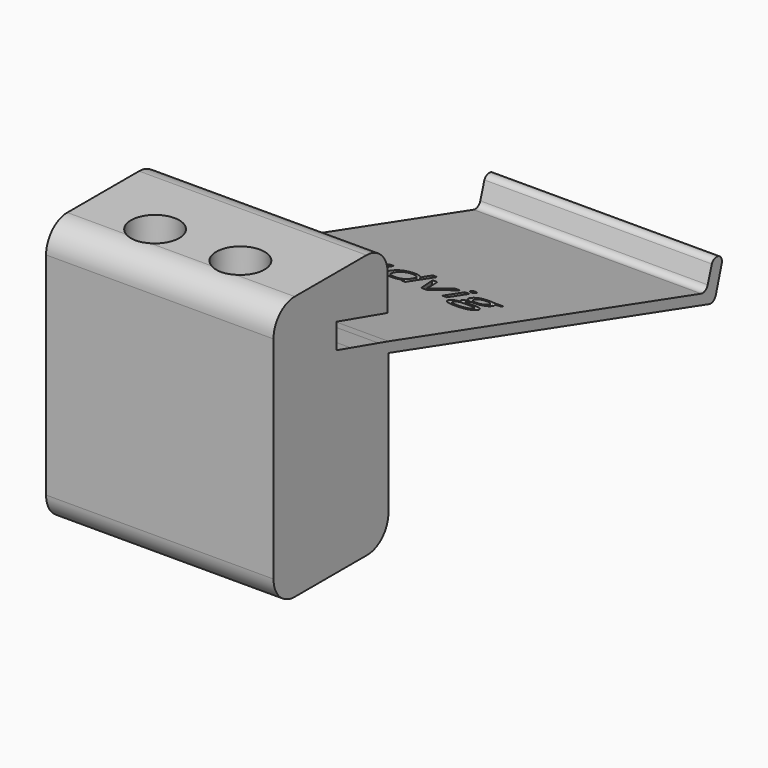
from build123d import *

# Parameters (mm, degrees)
F1_DEPTH  = 80
F4_DEPTH  = 22
F5_R      = 8.5
F6_DEPTH  = 22.5
F7_W      = 49.4286736109
F7_H      = 16.9561356306
F8_DEPTH  = 60.3
F9_W      = 1.5755122692
F9_H      = 10.3971667088
F10_DEPTH = 25


with BuildPart() as f1:
    # F0 (on Right) → F1 (new body)
    with BuildSketch(Plane.YZ):
        with BuildLine():
            ThreePointArc((-32.2318291664, 12.8581181365), (-34.9619750491, 19.4492733537), (-41.5531302664, 22.1794192365))
            Line((-41.5531302664, 22.1794192365), (-73.1118463473, 22.1794192365))
            ThreePointArc((-73.1118463473, 22.1794192365), (-79.7030015645, 19.4492733537), (-82.4331474473, 12.8581181365))
            Line((-82.4331474473, 12.8581181365), (-82.4331474473, -61.4992796635))
            ThreePointArc((-82.4331474473, -61.4992796635), (-81.2610502569, -66.0244459408), (-78.0395269394, -69.411587682))
            ThreePointArc((-78.0395269394, -69.411587682), (-76.5766946037, -70.1526882843), (-75.0066265464, -70.6259692164))
            ThreePointArc((-75.0066265464, -70.6259692164), (-74.0642204409, -70.7718002369), (-73.1118463473, -70.8205807635))
            Line((-73.1118463473, -70.8205807635), (-41.2218374732, -70.8205807635))
            ThreePointArc((-41.2218374732, -70.8205807635), (-34.6318795569, -68.0916319644), (-31.9005369883, -61.5026658346))
            Line((-31.9005369883, -61.5026658346), (-31.8690812334, -12.0527898285))
            Line((-31.8690812334, -12.0527898285), (109.1177060866, -54.2338658538))
            ThreePointArc((109.1177060866, -54.2338658538), (110.9069761748, -54.0507418606), (112.0426929702, -52.6560486304))
            Line((112.0426929702, -52.6560486304), (114.6341549506, -43.9942994883))
            ThreePointArc((114.6341549506, -43.9942994883), (114.6437769241, -42.6132673159), (113.9095705006, -41.4435308622))
            ThreePointArc((113.9095705006, -41.4435308622), (111.9034454417, -40.9732191466), (110.2978432915, -42.2646418492))
            Line((110.2978432915, -42.2646418492), (108.4831164642, -48.0129623561))
            ThreePointArc((108.4831164642, -48.0129623561), (107.3421845247, -49.382125377), (105.5685471657, -49.5568926134))
            Line((105.5685471657, -49.5568926134), (-31.8690812334, -8.4376702916))
            Line((-31.8690812334, -8.4376702916), (-36.2959507962, -7.1745254594))
            Line((-36.2959507962, -7.1745254594), (-48.491592755, -3.6946709262))
            Line((-48.491592755, -3.6946709262), (-54.7467279284, -1.9102199003))
            Line((-54.7467279284, -1.9102199003), (-54.7467279284, 6.9293941378))
            Line((-54.7467279284, 6.9293941378), (-50.4331474473, 5.6985747482))
            Line((-50.4331474473, 5.6985747482), (-46.4961274784, 4.5752015931))
            Line((-46.4961274784, 4.5752015931), (-32.2318291664, 0.5050851276))
            Line((-32.2318291664, 0.5050851276), (-32.2318291664, 12.8581181365))
        make_face()
    extrude(amount=F1_DEPTH)

    # F3 (on face) → F4 (cut)
    with BuildSketch(Plane(origin=(0, -54.7467279284, 0), x_dir=(-1, 0, 0), z_dir=(0, 1, 0))):
        Polygon((-71, 5.1884208806), (-71, 2.5095871187), (-71, 0), (-9, 0), (-9, 5.1884208806), (-69.0773031712, 5.1884208806), align=None)
    extrude(amount=-F4_DEPTH, mode=Mode.SUBTRACT)

    # F5 (on face) → F6 (cut)
    with BuildSketch(Plane(origin=(0, 0, 5.1884208806), x_dir=(1, 0, 0), z_dir=(0, 0, -1))):
        with Locations((55, 65.7467279284)):
            Circle(F5_R)
        with Locations((25, 65.7467279284)):
            Circle(F5_R)
    extrude(amount=-F6_DEPTH, mode=Mode.SUBTRACT)

    # F7 (on face) → F8 (cut)
    with BuildSketch(Plane.XY):
        with Locations((38.2213593278, -65.6192749739)):
            Rectangle(F7_W, F7_H)
    extrude(amount=-F8_DEPTH, mode=Mode.SUBTRACT)

    # F9 (on face) → F10 (cut)
    with BuildSketch(Plane(origin=(0, -4.9353020431, -16.4958423322), x_dir=(1, 0, 0), z_dir=(0, 0.286631123, 0.9580410217))):
        with BuildLine():
            Line((68.1775680531, 38.9351487613), (68.1775680531, 39.9308482301))
            Line((68.1775680531, 39.9308482301), (64.5833358245, 39.9308482301))
            add(Edge.make_bspline(
                [(63.1110363051, 40.1220953841), (63.9276312963, 40.1220953841), (64.5833358245, 39.9308482301)],
                knots=[0, 0, 0, 1, 1, 1], degree=2))
            add(Edge.make_bspline(
                [(60.2104544685, 39.1962163049), (61.2349927939, 40.1220953841), (63.1110363051, 40.1220953841)],
                knots=[0, 0, 0, 1, 1, 1], degree=2))
            add(Edge.make_bspline(
                [(59.1859161432, 36.5642911848), (59.1859161432, 38.2703372258), (60.2104544685, 39.1962163049)],
                knots=[0, 0, 0, 1, 1, 1], degree=2))
            add(Edge.make_bspline(
                [(59.6928728849, 34.741371883), (59.1859161432, 35.5382350249), (59.1859161432, 36.5642911848)],
                knots=[0, 0, 0, 1, 1, 1], degree=2))
            add(Edge.make_bspline(
                [(61.0073176104, 33.6136208078), (60.1998296266, 33.9445087411), (59.6928728849, 34.741371883)],
                knots=[0, 0, 0, 1, 1, 1], degree=2))
            add(Edge.make_bspline(
                [(60.048046171, 32.7879188094), (60.3516130822, 33.2159481542), (61.0073176104, 33.6136208078)],
                knots=[0, 0, 0, 1, 1, 1], degree=2))
            add(Edge.make_bspline(
                [(59.7444792598, 31.7922193406), (59.7444792598, 32.3598894646), (60.048046171, 32.7879188094)],
                knots=[0, 0, 0, 1, 1, 1], degree=2))
            add(Edge.make_bspline(
                [(60.0146538108, 30.908839629), (59.7444792598, 31.288298268), (59.7444792598, 31.7922193406)],
                knots=[0, 0, 0, 1, 1, 1], degree=2))
            add(Edge.make_bspline(
                [(60.6825010155, 30.3502765124), (60.2848283618, 30.52938099), (60.0146538108, 30.908839629)],
                knots=[0, 0, 0, 1, 1, 1], degree=2))
            add(Edge.make_bspline(
                [(58.9764549745, 29.4107369222), (59.5835887969, 30.1043873143), (60.6825010155, 30.3502765124)],
                knots=[0, 0, 0, 1, 1, 1], degree=2))
            add(Edge.make_bspline(
                [(58.3693211521, 27.7699577671), (58.3693211521, 28.7170865301), (58.9764549745, 29.4107369222)],
                knots=[0, 0, 0, 1, 1, 1], degree=2))
            add(Edge.make_bspline(
                [(59.4743047089, 25.6237397049), (58.3693211521, 26.3826569829), (58.3693211521, 27.7699577671)],
                knots=[0, 0, 0, 1, 1, 1], degree=2))
            add(Edge.make_bspline(
                [(62.619257909, 24.8648224269), (60.5792882656, 24.8648224269), (59.4743047089, 25.6237397049)],
                knots=[0, 0, 0, 1, 1, 1], degree=2))
            add(Edge.make_bspline(
                [(66.6597334971, 25.7709696568), (65.275468382, 24.8648224269), (62.619257909, 24.8648224269)],
                knots=[0, 0, 0, 1, 1, 1], degree=2))
            add(Edge.make_bspline(
                [(68.0439986122, 28.4044126115), (68.0439986122, 26.6771168868), (66.6597334971, 25.7709696568)],
                knots=[0, 0, 0, 1, 1, 1], degree=2))
            add(Edge.make_bspline(
                [(67.1393692168, 30.4732211114), (68.0439986122, 29.7613567046), (68.0439986122, 28.4044126115)],
                knots=[0, 0, 0, 1, 1, 1], degree=2))
            add(Edge.make_bspline(
                [(64.543872126, 31.1850855182), (66.2347398214, 31.1850855182), (67.1393692168, 30.4732211114)],
                knots=[0, 0, 0, 1, 1, 1], degree=2))
            Line((64.543872126, 31.1850855182), (62.7042566441, 31.1850855182))
            add(Edge.make_bspline(
                [(61.5006138412, 31.3884753487), (61.8512336236, 31.1850855182), (62.7042566441, 31.1850855182)],
                knots=[0, 0, 0, 1, 1, 1], degree=2))
            add(Edge.make_bspline(
                [(61.1499940587, 32.019894524), (61.1499940587, 31.5918651792), (61.5006138412, 31.3884753487)],
                knots=[0, 0, 0, 1, 1, 1], degree=2))
            add(Edge.make_bspline(
                [(62.1548005348, 33.3555889333), (61.1499940587, 32.8243468387), (61.1499940587, 32.019894524)],
                knots=[0, 0, 0, 1, 1, 1], degree=2))
            add(Edge.make_bspline(
                [(63.02603757, 33.2796972055), (62.5615801958, 33.2796972055), (62.1548005348, 33.3555889333)],
                knots=[0, 0, 0, 1, 1, 1], degree=2))
            add(Edge.make_bspline(
                [(65.8917092118, 34.1903979391), (64.8474390372, 33.2796972055), (63.02603757, 33.2796972055)],
                knots=[0, 0, 0, 1, 1, 1], degree=2))
            add(Edge.make_bspline(
                [(66.9359793863, 36.6310759052), (66.9359793863, 35.1010986728), (65.8917092118, 34.1903979391)],
                knots=[0, 0, 0, 1, 1, 1], degree=2))
            add(Edge.make_bspline(
                [(66.7265182176, 37.8392722118), (66.9359793863, 37.301958779), (66.9359793863, 36.6310759052)],
                knots=[0, 0, 0, 1, 1, 1], degree=2))
            add(Edge.make_bspline(
                [(66.2529538361, 38.7074735779), (66.5170570488, 38.3765856447), (66.7265182176, 37.8392722118)],
                knots=[0, 0, 0, 1, 1, 1], degree=2))
            Line((66.2529538361, 38.7074735779), (68.1775680531, 38.9351487613))
        make_face()
        with BuildLine():
            Line((58.4288015962, 28.3339321613), (58.4874711931, 28.3339321613))
            Line((58.4874711931, 28.3339321613), (59.9432890305, 28.3339321613))
            add(Edge.make_bspline(
                [(60.4851825232, 29.2589534666), (60.0703747901, 28.9041559893), (59.9432890305, 28.3339321613)],
                knots=[0, 0, 0, 0.6936273134, 0.6936273134, 0.6936273134], degree=2))
            add(Edge.make_bspline(
                [(62.1548005348, 29.770463712), (61.0832093382, 29.770463712), (60.4851825232, 29.2589534666)],
                knots=[0, 0, 0, 1, 1, 1], degree=2))
            Line((62.1548005348, 29.770463712), (64.0429867225, 29.770463712))
            add(Edge.make_bspline(
                [(66.0055468035, 29.4426114479), (65.4849295507, 29.770463712), (64.0429867225, 29.770463712)],
                knots=[0, 0, 0, 1, 1, 1], degree=2))
            add(Edge.make_bspline(
                [(66.5254195492, 28.3339321613), (66.5064764157, 29.1271572314), (66.0055468035, 29.4426114479)],
                knots=[0.0378159586, 0.0378159586, 0.0378159586, 1, 1, 1], degree=2))
            Line((66.5254195492, 28.3339321613), (67.9926872253, 28.3339321613))
            Line((67.9926872253, 28.3339321613), (68.0369660258, 28.3339321613))
            Line((68.0369660258, 28.3339321613), (68.0369660258, 28.2860677689))
            Line((68.0369660258, 28.2860677689), (68.0369660258, 28.1646177173))
            Line((68.0369660258, 28.1646177173), (68.034209311, 28.1332600862))
            Line((68.034209311, 28.1332600862), (66.5219728583, 28.1382272438))
            add(Edge.make_bspline(
                [(65.572963955, 26.6634563758), (66.4629576461, 27.2175766516), (66.5219728583, 28.1382272438)],
                knots=[0, 0, 0, 0.9336903028, 0.9336903028, 0.9336903028], degree=2))
            add(Edge.make_bspline(
                [(62.6374719236, 26.0699830644), (64.6197638538, 26.0699830644), (65.572963955, 26.6634563758)],
                knots=[0, 0, 0, 1, 1, 1], degree=2))
            add(Edge.make_bspline(
                [(60.5990201149, 26.5071194165), (61.3108845217, 26.0699830644), (62.6374719236, 26.0699830644)],
                knots=[0, 0, 0, 1, 1, 1], degree=2))
            add(Edge.make_bspline(
                [(59.8871557081, 27.7881717818), (59.8871557081, 26.9442557686), (60.5990201149, 26.5071194165)],
                knots=[0, 0, 0, 1, 1, 1], degree=2))
            add(Edge.make_bspline(
                [(59.9119054363, 28.1599389586), (59.8871557081, 27.9833208141), (59.8871557081, 27.7881717818)],
                knots=[0.7965653679, 0.7965653679, 0.7965653679, 1, 1, 1], degree=2))
            Line((59.9119054363, 28.1599389586), (58.4874711931, 28.1646177173))
            Line((58.4874711931, 28.1646177173), (58.3997890353, 28.1646177173))
            Line((58.3997890353, 28.1646177173), (58.3997890353, 28.180770576))
            Line((58.3997890353, 28.180770576), (58.417674154, 28.2701700926))
            Line((58.417674154, 28.2701700926), (58.4288015962, 28.3339321613))
        make_face(mode=Mode.SUBTRACT)
        with BuildLine():
            add(Edge.make_bspline(
                [(60.7401787286, 36.6007192141), (60.7401787286, 35.5109140029), (61.3564195583, 34.9508330517)],
                knots=[0, 0, 0, 1, 1, 1], degree=2))
            add(Edge.make_bspline(
                [(61.3382055437, 38.3750678101), (60.7401787286, 37.7785588296), (60.7401787286, 36.6007192141)],
                knots=[0, 0, 0, 1, 1, 1], degree=2))
            add(Edge.make_bspline(
                [(63.0472872538, 38.9715767906), (61.9362323587, 38.9715767906), (61.3382055437, 38.3750678101)],
                knots=[0, 0, 0, 1, 1, 1], degree=2))
            add(Edge.make_bspline(
                [(65.3786811318, 36.6310759052), (65.3786811318, 38.9715767906), (63.0472872538, 38.9715767906)],
                knots=[0, 0, 0, 1, 1, 1], degree=2))
            add(Edge.make_bspline(
                [(63.0746082758, 34.3907521005), (65.3786811318, 34.3907521005), (65.3786811318, 36.6310759052)],
                knots=[0, 0, 0, 1, 1, 1], degree=2))
            add(Edge.make_bspline(
                [(61.3564195583, 34.9508330517), (61.9726603881, 34.3907521005), (63.0746082758, 34.3907521005)],
                knots=[0, 0, 0, 1, 1, 1], degree=2))
        make_face(mode=Mode.SUBTRACT)
        with BuildLine():
            Line((40.1067357739, 30.9270536437), (40.191734509, 30.9270536437))
            Line((40.191734509, 30.9270536437), (40.4011956777, 29.5336815212))
            Line((40.4011956777, 29.5336815212), (41.682248043, 29.5336815212))
            Line((41.682248043, 29.5336815212), (41.682248043, 44.2961404132))
            Line((41.682248043, 44.2961404132), (40.1067357739, 44.2961404132))
            Line((40.1067357739, 44.2961404132), (40.1067357739, 40.064417671))
            Line((40.1067357739, 40.064417671), (40.1461994723, 39.332821415))
            Line((40.1461994723, 39.332821415), (40.2129841928, 38.5830111443))
            Line((40.2129841928, 38.5830111443), (40.0885217592, 38.5830111443))
            add(Edge.make_bspline(
                [(36.8433914784, 40.1220953841), (38.9592528495, 40.1220953841), (40.0885217592, 38.5830111443)],
                knots=[0, 0, 0, 1, 1, 1], degree=2))
            add(Edge.make_bspline(
                [(33.6741529254, 38.6983665706), (34.8125288424, 40.1220953841), (36.8433914784, 40.1220953841)],
                knots=[0, 0, 0, 1, 1, 1], degree=2))
            add(Edge.make_bspline(
                [(32.5357770084, 34.7034260191), (32.5357770084, 37.274637757), (33.6741529254, 38.6983665706)],
                knots=[0, 0, 0, 1, 1, 1], degree=2))
            add(Edge.make_bspline(
                [(33.6695994217, 30.7373243242), (32.5357770084, 32.1322142812), (32.5357770084, 34.7034260191)],
                knots=[0, 0, 0, 1, 1, 1], degree=2))
            add(Edge.make_bspline(
                [(36.8433914784, 29.3424343672), (34.8034218351, 29.3424343672), (33.6695994217, 30.7373243242)],
                knots=[0, 0, 0, 1, 1, 1], degree=2))
            add(Edge.make_bspline(
                [(40.1067357739, 30.9270536437), (39.0169305626, 29.3424343672), (36.8433914784, 29.3424343672)],
                knots=[0, 0, 0, 1, 1, 1], degree=2))
        make_face()
        with BuildLine():
            add(Edge.make_bspline(
                [(37.0437456398, 30.6629504309), (38.6556859383, 30.6629504309), (39.3812108561, 31.5402588043)],
                knots=[0, 0, 0, 1, 1, 1], degree=2))
            add(Edge.make_bspline(
                [(34.8990454121, 31.6783817489), (35.6291238336, 30.6629504309), (37.0437456398, 30.6629504309)],
                knots=[0, 0, 0, 1, 1, 1], degree=2))
            add(Edge.make_bspline(
                [(34.1689669907, 34.6852120044), (34.1689669907, 32.6938130669), (34.8990454121, 31.6783817489)],
                knots=[0, 0, 0, 1, 1, 1], degree=2))
            add(Edge.make_bspline(
                [(34.9035989158, 37.7254346201), (34.1689669907, 36.6492899199), (34.1689669907, 34.6852120044)],
                knots=[0, 0, 0, 1, 1, 1], degree=2))
            add(Edge.make_bspline(
                [(37.0255316251, 38.8015793204), (35.6382308409, 38.8015793204), (34.9035989158, 37.7254346201)],
                knots=[0, 0, 0, 1, 1, 1], degree=2))
            add(Edge.make_bspline(
                [(39.3721038487, 37.8574862265), (38.6374719236, 38.8015793204), (37.0255316251, 38.8015793204)],
                knots=[0, 0, 0, 1, 1, 1], degree=2))
            add(Edge.make_bspline(
                [(40.1067357739, 34.7034260191), (40.1067357739, 36.9133931327), (39.3721038487, 37.8574862265)],
                knots=[0, 0, 0, 1, 1, 1], degree=2))
            Line((40.1067357739, 34.7034260191), (40.1067357739, 34.3725380859))
            add(Edge.make_bspline(
                [(39.3812108561, 31.5402588043), (40.1067357739, 32.4175671777), (40.1067357739, 34.3725380859)],
                knots=[0, 0, 0, 1, 1, 1], degree=2))
        make_face(mode=Mode.SUBTRACT)
        with BuildLine():
            Line((22.6728880633, 33.185591463), (22.6728880633, 39.9308482301))
            Line((22.6728880633, 39.9308482301), (21.0791617794, 39.9308482301))
            Line((21.0791617794, 39.9308482301), (21.0791617794, 33.1279137499))
            add(Edge.make_bspline(
                [(22.0217370387, 30.2440280935), (21.0791617794, 31.1456218197), (21.0791617794, 33.1279137499)],
                knots=[0, 0, 0, 1, 1, 1], degree=2))
            add(Edge.make_bspline(
                [(24.8616054931, 29.3424343672), (22.964312298, 29.3424343672), (22.0217370387, 30.2440280935)],
                knots=[0, 0, 0, 1, 1, 1], degree=2))
            add(Edge.make_bspline(
                [(26.8226477395, 29.7507318627), (25.9635533807, 29.3424343672), (24.8616054931, 29.3424343672)],
                knots=[0, 0, 0, 1, 1, 1], degree=2))
            add(Edge.make_bspline(
                [(28.164413487, 30.9270536437), (27.6817420982, 30.1590293583), (26.8226477395, 29.7507318627)],
                knots=[0, 0, 0, 1, 1, 1], degree=2))
            Line((28.164413487, 30.9270536437), (28.2494122221, 30.9270536437))
            Line((28.2494122221, 30.9270536437), (28.4770874055, 29.5336815212))
            Line((28.4770874055, 29.5336815212), (29.7763537855, 29.5336815212))
            Line((29.7763537855, 29.5336815212), (29.7763537855, 39.9308482301))
            Line((29.7763537855, 39.9308482301), (28.2008415163, 39.9308482301))
            Line((28.2008415163, 39.9308482301), (28.2008415163, 34.4666438283))
            add(Edge.make_bspline(
                [(27.4479955765, 31.5539193153), (28.2008415163, 32.4448881997), (28.2008415163, 34.4666438283)],
                knots=[0, 0, 0, 1, 1, 1], degree=2))
            add(Edge.make_bspline(
                [(25.0619596545, 30.6629504309), (26.6951496368, 30.6629504309), (27.4479955765, 31.5539193153)],
                knots=[0, 0, 0, 1, 1, 1], degree=2))
            add(Edge.make_bspline(
                [(23.2511830291, 31.288298268), (23.829477995, 30.6629504309), (25.0619596545, 30.6629504309)],
                knots=[0, 0, 0, 1, 1, 1], degree=2))
            add(Edge.make_bspline(
                [(22.6728880633, 33.185591463), (22.6728880633, 31.9136461051), (23.2511830291, 31.288298268)],
                knots=[0, 0, 0, 1, 1, 1], degree=2))
        make_face()
        with BuildLine():
            Line((43.3518660547, 39.9308482301), (47.2982359004, 29.5336815212))
            Line((47.2982359004, 29.5336815212), (49.1378513823, 29.5336815212))
            Line((49.1378513823, 29.5336815212), (53.084221228, 39.9308482301))
            Line((53.084221228, 39.9308482301), (51.3963892016, 39.9308482301))
            add(Edge.make_bspline(
                [(48.9071405297, 33.0383615111), (49.4626679773, 34.6184272839), (51.3963892016, 39.9308482301)],
                knots=[0, 0, 0, 1, 1, 1], degree=2))
            add(Edge.make_bspline(
                [(48.2484003324, 30.9574103348), (48.3516130822, 31.4582957383), (48.9071405297, 33.0383615111)],
                knots=[0, 0, 0, 1, 1, 1], degree=2))
            Line((48.2484003324, 30.9574103348), (48.1725086046, 30.9574103348))
            add(Edge.make_bspline(
                [(47.2800218857, 33.7654042635), (48.0389391637, 31.6009721865), (48.1725086046, 30.9574103348)],
                knots=[0, 0, 0, 1, 1, 1], degree=2))
            Line((47.2800218857, 33.7654042635), (45.039698081, 39.9308482301))
            Line((45.039698081, 39.9308482301), (43.3518660547, 39.9308482301))
        make_face()
        Polygon((11.343770937, 43.4036536943), (11.343770937, 29.5336815212), (19.0756201655, 29.5336815212), (19.0756201655, 30.9938383641), (12.9557112355, 30.9938383641), (12.9557112355, 43.4036536943), align=None)
        with Locations((55.5415953742, 34.7322648756)):
            Rectangle(F9_W, F9_H)
        with BuildLine():
            add(Edge.make_bspline(
                [(54.6202697987, 42.7479491661), (54.6202697987, 43.288298268), (54.885890846, 43.5402588043)],
                knots=[0, 0, 0, 1, 1, 1], degree=2))
            add(Edge.make_bspline(
                [(54.885890846, 41.9556395278), (54.6202697987, 42.2167070714), (54.6202697987, 42.7479491661)],
                knots=[0, 0, 0, 1, 1, 1], degree=2))
            add(Edge.make_bspline(
                [(55.5522202161, 41.6945719842), (55.1515118933, 41.6945719842), (54.885890846, 41.9556395278)],
                knots=[0, 0, 0, 1, 1, 1], degree=2))
            add(Edge.make_bspline(
                [(56.2064069097, 41.9556395278), (55.9316788551, 41.6945719842), (55.5522202161, 41.6945719842)],
                knots=[0, 0, 0, 1, 1, 1], degree=2))
            add(Edge.make_bspline(
                [(56.4811349644, 42.7479491661), (56.4811349644, 42.2167070714), (56.2064069097, 41.9556395278)],
                knots=[0, 0, 0, 1, 1, 1], degree=2))
            add(Edge.make_bspline(
                [(56.2064069097, 43.5357053006), (56.4811349644, 43.2791912607), (56.4811349644, 42.7479491661)],
                knots=[0, 0, 0, 1, 1, 1], degree=2))
            add(Edge.make_bspline(
                [(55.5522202161, 43.7922193406), (55.9316788551, 43.7922193406), (56.2064069097, 43.5357053006)],
                knots=[0, 0, 0, 1, 1, 1], degree=2))
            add(Edge.make_bspline(
                [(54.885890846, 43.5402588043), (55.1515118933, 43.7922193406), (55.5522202161, 43.7922193406)],
                knots=[0, 0, 0, 1, 1, 1], degree=2))
        make_face()
        with BuildLine():
            Line((67.9926872253, 28.3339321613), (66.5254195492, 28.3339321613))
            add(Edge.make_bspline(
                [(66.5261640562, 28.2708431706), (66.5261640562, 28.3027566636), (66.5254195492, 28.3339321613)],
                knots=[0, 0, 0, 0.0378159586, 0.0378159586, 0.0378159586], degree=2))
            add(Edge.make_bspline(
                [(66.5219728583, 28.1382272438), (66.5261640562, 28.2036108745), (66.5261640562, 28.2708431706)],
                knots=[0.9336903028, 0.9336903028, 0.9336903028, 1, 1, 1], degree=2))
            Line((66.5219728583, 28.1382272438), (68.034209311, 28.1332600862))
            Line((68.034209311, 28.1332600862), (68.0369660258, 28.1646177173))
            Line((68.0369660258, 28.1646177173), (68.0369660258, 28.2860677689))
            Line((68.0369660258, 28.2860677689), (68.0369660258, 28.3339321613))
            Line((68.0369660258, 28.3339321613), (67.9926872253, 28.3339321613))
        make_face()
        with BuildLine():
            Line((59.9432890305, 28.3339321613), (58.4874711931, 28.3339321613))
            Line((58.4874711931, 28.3339321613), (58.4288015962, 28.3339321613))
            Line((58.4288015962, 28.3339321613), (58.417674154, 28.2701700926))
            Line((58.417674154, 28.2701700926), (58.3997890353, 28.180770576))
            Line((58.3997890353, 28.180770576), (58.3997890353, 28.1646177173))
            Line((58.3997890353, 28.1646177173), (58.4874711931, 28.1646177173))
            Line((58.4874711931, 28.1646177173), (59.9119054363, 28.1599389586))
            add(Edge.make_bspline(
                [(59.9432890305, 28.3339321613), (59.9244288146, 28.2493078532), (59.9119054363, 28.1599389586)],
                knots=[0.6936273134, 0.6936273134, 0.6936273134, 0.7965653679, 0.7965653679, 0.7965653679], degree=2))
        make_face()
    extrude(amount=-F10_DEPTH, mode=Mode.SUBTRACT)


with BuildPart() as f1b:
    # F0 (on Right) → F1, piece 2 (new body)
    with BuildSketch(Plane.YZ):
        with BuildLine():
            ThreePointArc((113.8705675473, -41.4095936453), (113.8901579421, -41.4264600631), (113.9095705006, -41.4435308622))
            ThreePointArc((113.9095705006, -41.4435308622), (113.9290391903, -41.4595818344), (113.9483344197, -41.4758409153))
            Line((113.9483344197, -41.4758409153), (113.8705675473, -41.4095936453))
        make_face()
    extrude(amount=F1_DEPTH)


solid = Compound([f1.part, f1b.part])
